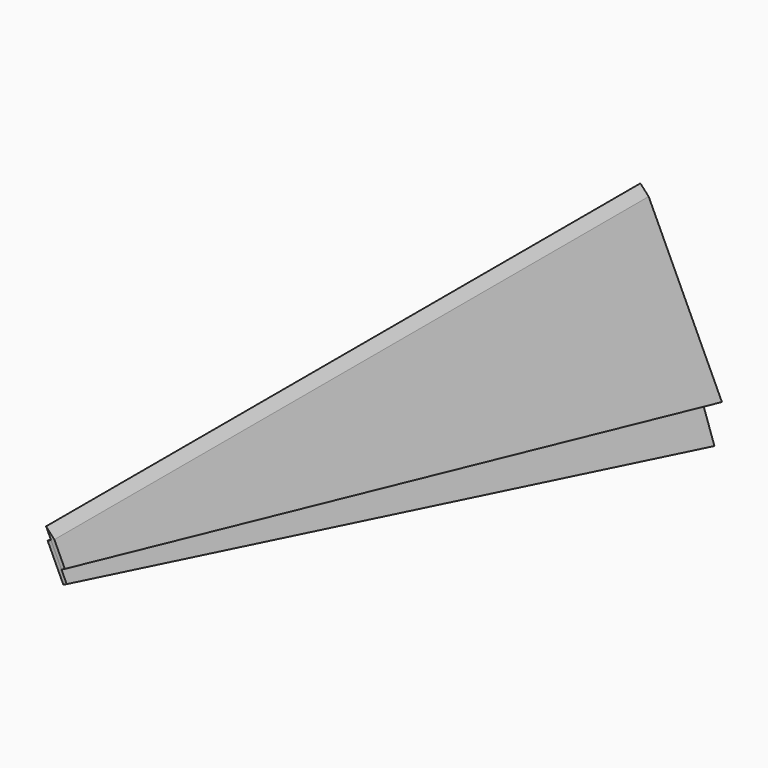
from build123d import *

# Parameters (mm, degrees)
F3_DEPTH    = 1.5
F4_DEPTH    = 1.5
F5_T1_DEPTH = 325.9542136725


# Not quite as in the source:
# - a fillet or chamfer that OpenCascade refuses, or shapes differently, is made with other operations: its cross-section is extruded or revolved along the edge and cut away or added


with BuildPart() as f3:
    # F2 (on line) → F3 (new body)
    with BuildSketch(Plane(origin=(1.6427876097, 0, 0.7660444431), x_dir=(0, -1, 0), z_dir=(-0.906307787, 0, -0.4226182617))):
        Polygon((150, -5.8452365235), (150, -0.8452365235), (-150, -0.8452365235), (-150, -12.8946734447), align=None)
        Polygon((-143.2140751153, -74.4880515465), (-150, -12.8946734447), (-150, -75.8452365235), align=None)
        Polygon((150, -15.8452365235), (150, -5.8452365235), (-150, -12.8946734447), (-143.2140751153, -74.4880515465), align=None)
    extrude(amount=-F3_DEPTH)

    # F5: chamfer of 1.6 x 5 on 1 edges, made by hand

    # F5_s2 → F5_t1 (cut)
    with BuildSketch(Plane.XZ.offset(-162.9771068363)):
        Polygon((1.9093692213, -0.0422618262), (5.4725529893, -3.8976115426), (3.3594616806, 0.6339273926), align=None)
    extrude(amount=F5_T1_DEPTH, mode=Mode.SUBTRACT)


with BuildPart() as f4:
    # F2 (on line) → F4 (new body)
    with BuildSketch(Plane(origin=(1.6427876097, 0, 0.7660444431), x_dir=(0, -1, 0), z_dir=(-0.906307787, 0, -0.4226182617))):
        Polygon((150, -20.8452365235), (150, -15.8452365235), (-143.2140751153, -74.4880515465), (-141.7867242303, -87.4435976565), align=None)
        Polygon((150, -15.8452365235), (150, -5.8452365235), (-150, -12.8946734447), (-143.2140751153, -74.4880515465), align=None)
    extrude(amount=F4_DEPTH)


solid = Compound([f3.part, f4.part])
